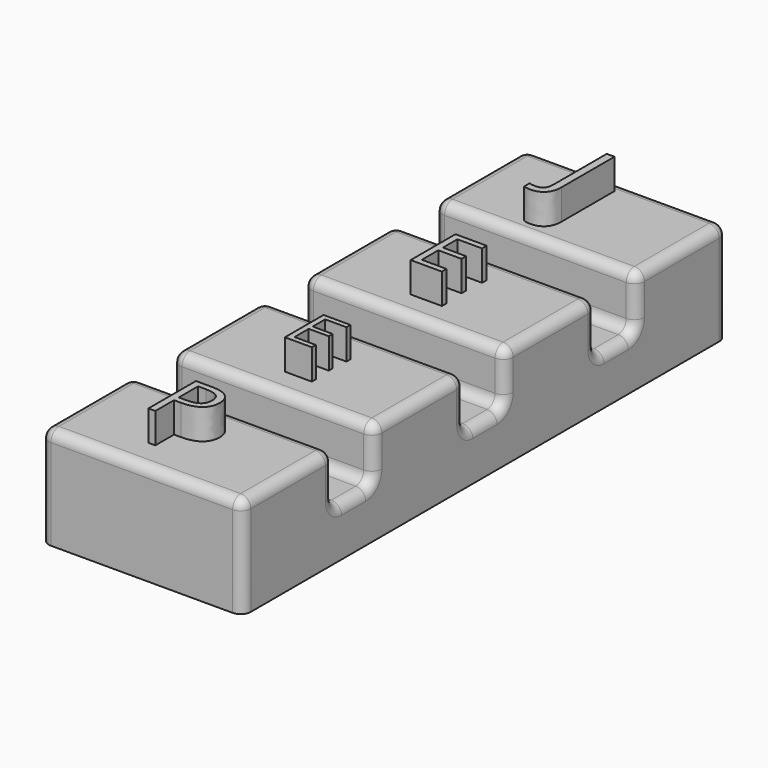
from build123d import *

# Parameters (mm, degrees)
F0_W          = 25.4
F0_H          = 76.2
F1_DEPTH      = 12.7
F2_W          = 6.35
F2_H          = 12.8523909211
F2_H_2        = 13.0550377156
F3_DEPTH      = 25.401
F4_R          = 1.27
F5_T          = -2.54
F6_TEXT_SIZE  = 11.7725382249
F7_DEPTH      = 3.81
F8_TEXT_SIZE  = 9.8765885923
F9_DEPTH      = 3.81
F10_TEXT_SIZE = 8.5168757424
F11_DEPTH     = 3.81
F12_TEXT_SIZE = 10.4679182793
F13_DEPTH     = 3.81


# Not quite as in the source:
# - Text() gives the source's letters only with a copy of the font that has no kerning and outlines rounded to 1/6400 em; it was checked with that copy


with BuildPart() as f1:
    # F0 (on Top) → F1 (new body)
    with BuildSketch(Plane.XY):
        Rectangle(F0_W, F0_H)
    extrude(amount=F1_DEPTH)

    # F2 (on face) → F3 (cut, through all)
    with BuildSketch(Plane.YZ.offset(12.7)):
        with Locations((0, 12.7)):
            Rectangle(F2_W, F2_H)
        with Locations((20.6375, 12.7)):
            Rectangle(F2_W, F2_H_2)
        with Locations((-20.6502, 12.7)):
            Rectangle(F2_W, F2_H_2)
    extrude(amount=-F3_DEPTH, mode=Mode.SUBTRACT)

    # F4
    f4_edges = [f1.edges().sort_by_distance(p)[0] for p in [
        (12.7, -30.9626, 12.7),
        (0, -38.1, 12.7),
        (-12.7, -30.9626, 12.7),
        (0, -23.8252, 12.7),
        (12.7, -10.3251, 12.7),
        (0, -17.4752, 12.7),
        (-12.7, -10.3251, 12.7),
        (0, -3.175, 12.7),
        (12.7, 10.31875, 12.7),
        (0, 3.175, 12.7),
        (-12.7, 10.31875, 12.7),
        (0, 17.4625, 12.7),
        (12.7, 30.95625, 12.7),
        (0, 23.8125, 12.7),
        (-12.7, 30.95625, 12.7),
        (0, 38.1, 12.7),
        (12.7, -20.6502, 6.172481),
        (0, -17.4752, 6.172481),
        (-12.7, -20.6502, 6.172481),
        (0, -23.8252, 6.172481),
        (12.7, 0, 6.273805),
        (0, 3.175, 6.273805),
        (-12.7, 0, 6.273805),
        (0, -3.175, 6.273805),
        (12.7, 20.6375, 6.172481),
        (0, 23.8125, 6.172481),
        (-12.7, 20.6375, 6.172481),
        (0, 17.4625, 6.172481),
        (12.7, 38.1, 6.35),
        (-12.7, 38.1, 6.35),
        (12.7, -38.1, 6.35),
        (-12.7, -38.1, 6.35),
        (12.7, 23.8125, 9.436241),
        (12.7, 17.4625, 9.436241),
        (12.7, 3.175, 9.486902),
        (12.7, -3.175, 9.486902),
        (12.7, -17.4752, 9.436241),
        (12.7, -23.8252, 9.436241),
        (-12.7, -23.8252, 9.436241),
        (-12.7, -17.4752, 9.436241),
        (-12.7, -3.175, 9.486902),
        (-12.7, 3.175, 9.486902),
        (-12.7, 17.4625, 9.436241),
        (-12.7, 23.8125, 9.436241),
    ]]
    fillet(f4_edges, radius=F4_R)

    # F5
    f5_openings = [f1.faces().sort_by_distance(p)[0] for p in [
        (0, 0, 0),
    ]]
    offset(amount=F5_T, openings=f5_openings)

    # F6 (on face) → F7 (join)
    with BuildSketch(Plane.XY.offset(12.7)):
        with Locations((-2.1563800983, 27.9607363045)):
            Text('J', F6_TEXT_SIZE, font='Open Sans', text_align=(TextAlign.LEFT, TextAlign.BOTTOM))
    extrude(amount=F7_DEPTH)

    # F8 (on face) → F9 (join)
    with BuildSketch(Plane.XY.offset(12.7)):
        with Locations((-2.959132893, 6.678877864)):
            Text('E', F8_TEXT_SIZE, font='Open Sans', text_align=(TextAlign.LEFT, TextAlign.BOTTOM))
    extrude(amount=F9_DEPTH)

    # F10 (on face) → F11 (join)
    with BuildSketch(Plane.XY.offset(12.7)):
        with Locations((-2.2103954434, -13.8702010736)):
            Text('E', F10_TEXT_SIZE, font='Open Sans', text_align=(TextAlign.LEFT, TextAlign.BOTTOM))
    extrude(amount=F11_DEPTH)

    # F12 (on face) → F13 (join)
    with BuildSketch(Plane.XY.offset(12.7)):
        with Locations((-3.4169199062, -34.0647194535)):
            Text('P', F12_TEXT_SIZE, font='Open Sans', text_align=(TextAlign.LEFT, TextAlign.BOTTOM))
    extrude(amount=F13_DEPTH)


solid = f1.part
